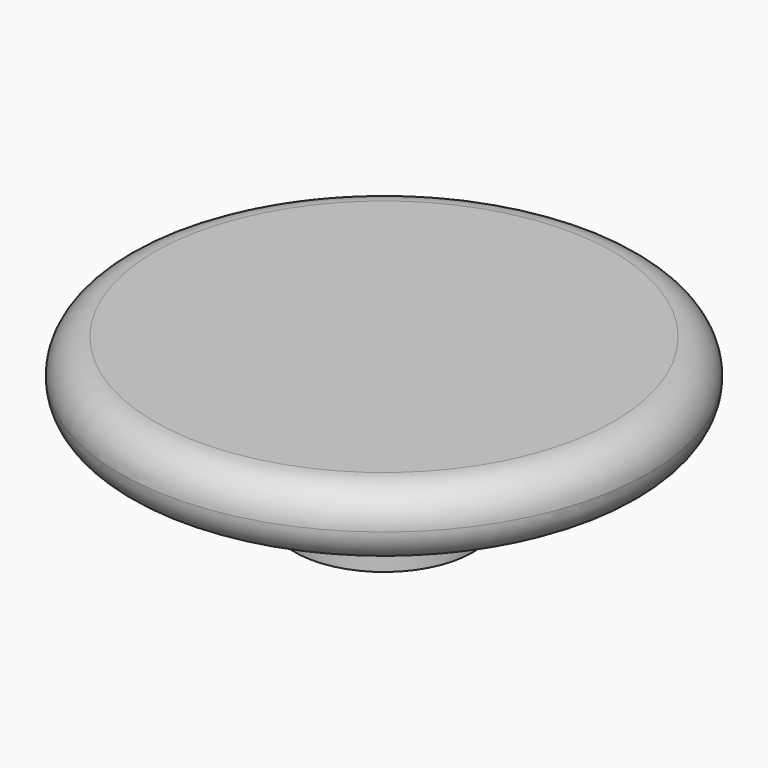
from build123d import *

# Parameters (mm, degrees)
F0_R     = 11.5
F1_DEPTH = 3
F2_R     = 1.5
F3_R     = 1.49999
F4_R     = 3.875
F5_DEPTH = 4


# Not quite as in the source:
# - a fillet or chamfer is up to 0.001 mm smaller than in the source, because OpenCascade refuses the exact size


with BuildPart() as f1:
    # F0 (on Top) → F1 (new body)
    with BuildSketch(Plane.XY):
        Circle(F0_R)
    extrude(amount=F1_DEPTH)

    # F2
    f2_edges = [f1.edges().sort_by_distance(p)[0] for p in [
        (-11.5, 0, 3),
    ]]
    fillet(f2_edges, radius=F2_R)

    # F3 (radius 1.5 in the source; OpenCascade refuses exactly that, so slightly less here)
    f3_edges = [f1.edges().sort_by_distance(p)[0] for p in [
        (-11.5, 0, 0),
    ]]
    fillet(f3_edges, radius=F3_R)

    # F4 (on face) → F5 (join)
    with BuildSketch(Plane(origin=(0, 0, 0), x_dir=(1, 0, 0), z_dir=(0, 0, -1))):
        Circle(F4_R)
    extrude(amount=F5_DEPTH)


solid = f1.part
